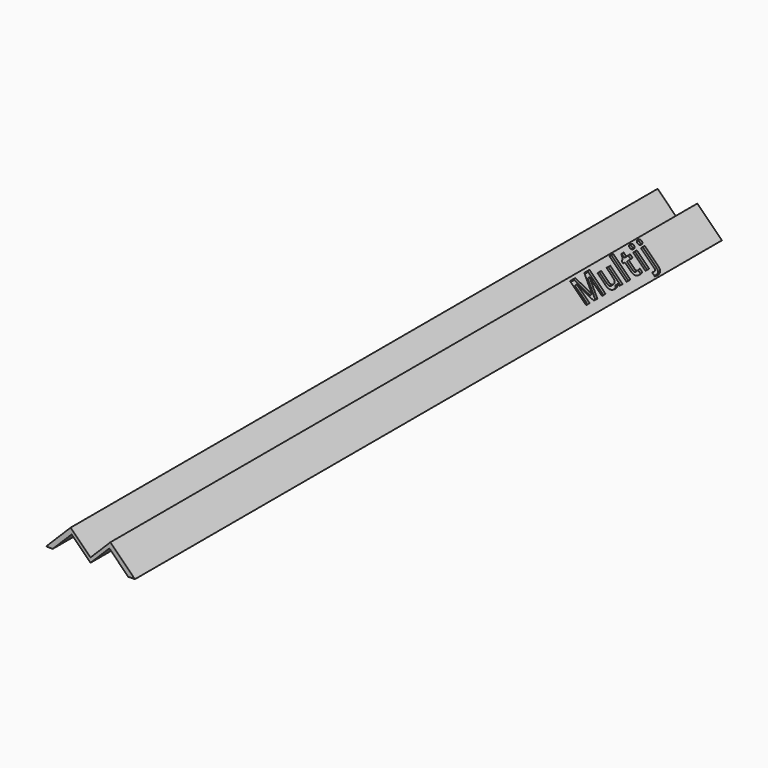
from build123d import *

# Parameters (mm, degrees)
F1_DEPTH     = 110
F2_TEXT_SIZE = 4.7737893409
F3_DEPTH     = 0.4


# Not quite as in the source:
# - Text() gives the source's letters only with a copy of the font that has no kerning and outlines rounded to 1/6400 em; it was checked with that copy


with BuildPart() as f1:
    # F0 (on Front) → F1 (new body)
    with BuildSketch(Plane.XZ):
        Polygon((-2.8284271247, 2.8284271247), (0, 0), (2.8284271247, 2.8284271247), (5.6568542495, 0), (6.6568542495, 0), (2.9784271247, 3.6784271247), (0, 0.7), (-2.9784271247, 3.6784271247), (-6.6568542495, 0), (-5.6568542495, 0), align=None)
    extrude(amount=F1_DEPTH)

    # F2 (on face) → F3 (cut)
    with BuildSketch(Plane(origin=(3.3284271247, 0, 3.3284271247), x_dir=(0, 1, 0), z_dir=(0.7071067812, 0, 0.7071067812))):
        with Locations((-24.6537681669, -3.3258210169)):
            Text('Multij', F2_TEXT_SIZE, font='Open Sans', font_style=FontStyle.BOLD, text_align=(TextAlign.LEFT, TextAlign.BOTTOM))
    extrude(amount=-F3_DEPTH, mode=Mode.SUBTRACT)


solid = f1.part
